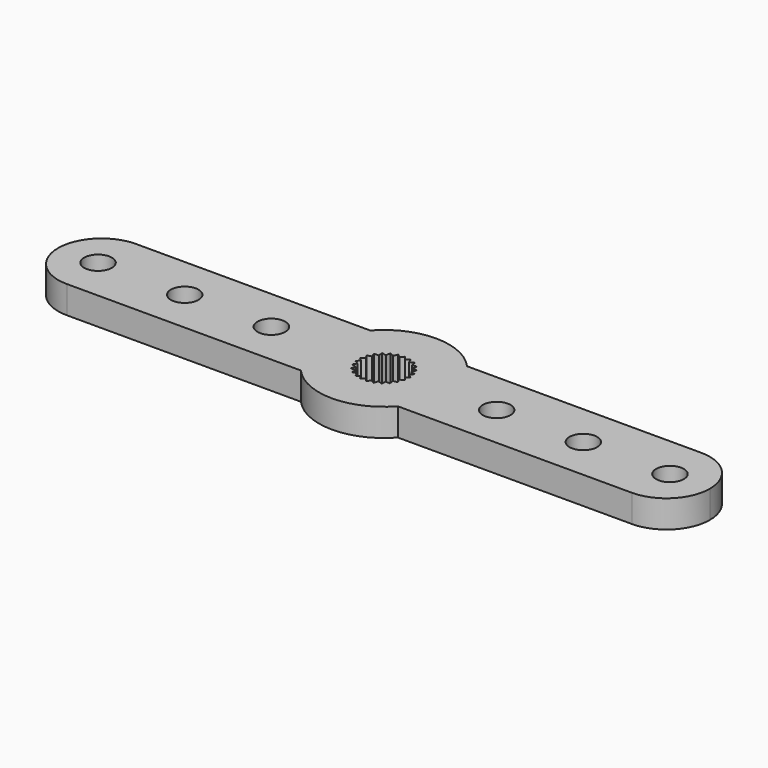
from build123d import *

# Parameters (mm, degrees)
F0_R     = 1.6
F1_DEPTH = 3.175


with BuildPart() as f1:
    # F0 (on Top) → F1 (new body)
    with BuildSketch(Plane.XY):
        with BuildLine():
            ThreePointArc((5.5901699437, 5), (0, 7.5), (-5.5901699437, 5))
            Line((-5.5901699437, 5), (-32.6, 5))
            ThreePointArc((-32.6, 5), (-36.1355339059, 3.5355339059), (-37.6, 0))
            ThreePointArc((-37.6, 0), (-36.1355339059, -3.5355339059), (-32.6, -5))
            Line((-32.6, -5), (-5.5901699437, -5))
            ThreePointArc((-5.5901699437, -5), (0, -7.5), (5.5901699437, -5))
            Line((5.5901699437, -5), (32.6, -5))
            ThreePointArc((32.6, -5), (36.1355339059, -3.5355339059), (37.6, 0))
            ThreePointArc((37.6, 0), (36.1355339059, 3.5355339059), (32.6, 5))
            Line((32.6, 5), (5.5901699437, 5))
        make_face()
        with Locations((-33, 0)):
            Circle(F0_R, mode=Mode.SUBTRACT)
        with Locations((-23, 0)):
            Circle(F0_R, mode=Mode.SUBTRACT)
        with Locations((-13, 0)):
            Circle(F0_R, mode=Mode.SUBTRACT)
        Polygon((-2.3131272616, 1.150841372), (-2.4811892868, 1.651717782), (-1.9542535042, 1.6899369317), (-1.992472654, 2.2168727143), (-1.4725868119, 2.1228475389), (-1.3785616365, 2.6427333809), (-0.8983920744, 2.4223718279), (-0.6780305213, 2.90254139), (-0.2677480588, 2.5696895861), (0.0651037451, 2.9799720486), (0.379719552, 2.555544297), (0.8041473037, 2.8701601039), (1.0033279869, 2.380824761), (1.4926633298, 2.5800054442), (1.5638936344, 2.0565092492), (2.0873898293, 2.1277395538), (2.0261940932, 1.6029756981), (2.5509579489, 1.5417799619), (2.3611813253, 1.0487212884), (2.8542399989, 0.8589446648), (2.547806851, 0.4285718633), (2.9781796525, 0.1221387154), (2.574344302, -0.2185063082), (2.9149893256, -0.6223416587), (2.4391262327, -0.8518549247), (2.6686394987, -1.3277180175), (2.1506488918, -1.4316783634), (2.2546092377, -1.9496689703), (1.7270383715, -1.9215441851), (1.6989135863, -2.4491150513), (1.1949116786, -2.2906723188), (1.0364689461, -2.7946742265), (0.5877042905, -2.5158690862), (0.3088991502, -2.9646337418), (-0.0564307197, -2.5829845462), (-0.4380799154, -2.9483144161), (-0.6970199802, -2.4878015876), (-1.1575328087, -2.7467416524), (-1.2938129119, -2.2363009057), (-1.8042536586, -2.3725810089), (-1.80931082, -1.8442852134), (-2.3376066155, -1.8493423749), (-2.2111230752, -1.3363862984), (-2.7240791517, -1.209902758), (-2.4740023355, -0.7445173173), (-2.9393877762, -0.4944405012), (-2.5814309304, -0.105867575), (-2.9700038565, 0.2520892708), (-2.5266587261, 0.5394342163), (-2.8140036716, 0.9827793468), align=None, mode=Mode.SUBTRACT)
        with Locations((13, 0)):
            Circle(F0_R, mode=Mode.SUBTRACT)
        with Locations((23, 0)):
            Circle(F0_R, mode=Mode.SUBTRACT)
        with Locations((33, 0)):
            Circle(F0_R, mode=Mode.SUBTRACT)
    extrude(amount=F1_DEPTH)


solid = f1.part
